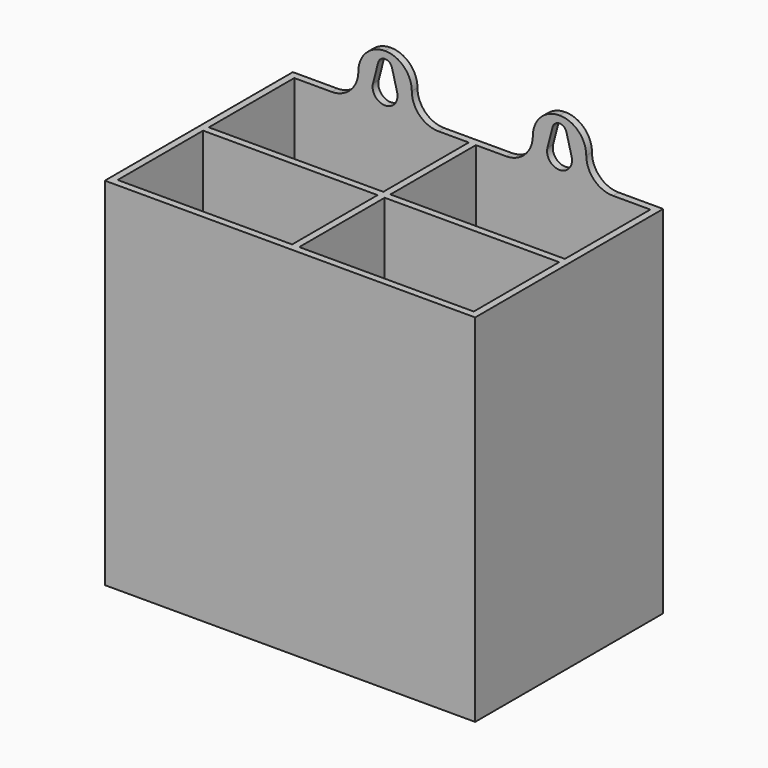
from build123d import *

# Parameters (mm, degrees)
F1_DEPTH  = 2
F2_W      = 104
F2_H      = 66
F2_W_2    = 49
F2_H_2    = 30
F3_DEPTH  = 100
F4_W      = 15
F4_H      = 2
F5_DEPTH  = 15
F7_DEPTH  = 2
F8_R      = 7.49999
F9_W      = 104
F9_H      = 66
F10_DEPTH = 2


# Not quite as in the source:
# - a fillet or chamfer is up to 0.001 mm smaller than in the source, because OpenCascade refuses the exact size


with BuildPart() as f1:
    # F0 (on Top) → F1 (new body)
    with BuildSketch(Plane.XY):
        Polygon((104, 0), (0, 0), (0, -34), (0, -66), (104, -66), (104, -34), align=None)
    extrude(amount=F1_DEPTH)

    # F2 (on face) → F3 (join)
    with BuildSketch(Plane.XY.offset(2)):
        with Locations((52, -33)):
            Rectangle(F2_W, F2_H)
        with Locations((26.5, -49)):
            Rectangle(F2_W_2, F2_H_2, mode=Mode.SUBTRACT)
        with Locations((77.5, -49)):
            Rectangle(F2_W_2, F2_H_2, mode=Mode.SUBTRACT)
        with Locations((26.5, -17)):
            Rectangle(F2_W_2, F2_H_2, mode=Mode.SUBTRACT)
        with Locations((77.5, -17)):
            Rectangle(F2_W_2, F2_H_2, mode=Mode.SUBTRACT)
    extrude(amount=F3_DEPTH)

    # F4 (on face) → F5 (join)
    with BuildSketch(Plane.XY.offset(102)):
        with Locations((27.5, -1)):
            Rectangle(F4_W, F4_H)
        with Locations((76.5, -1)):
            Rectangle(F4_W, F4_H)
    extrude(amount=F5_DEPTH)

    # F6 (on face) → F7 (cut, through all)
    with BuildSketch(Plane.XZ.offset(2)):
        with BuildLine():
            Line((79.8888604279, 107.875), (78.4364916731, 113.5))
            ThreePointArc((78.4364916731, 113.5), (76.5, 115), (74.5635083269, 113.5))
            Line((74.5635083269, 113.5), (73.1111395721, 107.875))
            ThreePointArc((73.1111395721, 107.875), (76.5, 103.5), (79.8888604279, 107.875))
        make_face()
        with BuildLine():
            Line((30.8888604279, 107.875), (29.4364916731, 113.5))
            ThreePointArc((29.4364916731, 113.5), (27.5, 115), (25.5635083269, 113.5))
            Line((25.5635083269, 113.5), (24.1111395721, 107.875))
            ThreePointArc((24.1111395721, 107.875), (27.5, 103.5), (30.8888604279, 107.875))
        make_face()
    extrude(amount=-F7_DEPTH, mode=Mode.SUBTRACT)

    # F8 (radius 7.5 in the source; OpenCascade refuses exactly that, so slightly less here)
    f8_edges = [f1.edges().sort_by_distance(p)[0] for p in [
        (84, -1, 102),
        (84, -1, 117),
        (69, -1, 117),
        (69, -1, 102),
        (35, -1, 102),
        (35, -1, 117),
        (20, -1, 117),
        (20, -1, 102),
    ]]
    fillet(f8_edges, radius=F8_R)

    # F9 (on face) → F10 (cut)
    with BuildSketch(Plane(origin=(0, 0, 0), x_dir=(1, 0, 0), z_dir=(0, 0, -1))):
        with Locations((52, 33)):
            Rectangle(F9_W, F9_H)
    extrude(amount=-F10_DEPTH, mode=Mode.SUBTRACT)


solid = f1.part
